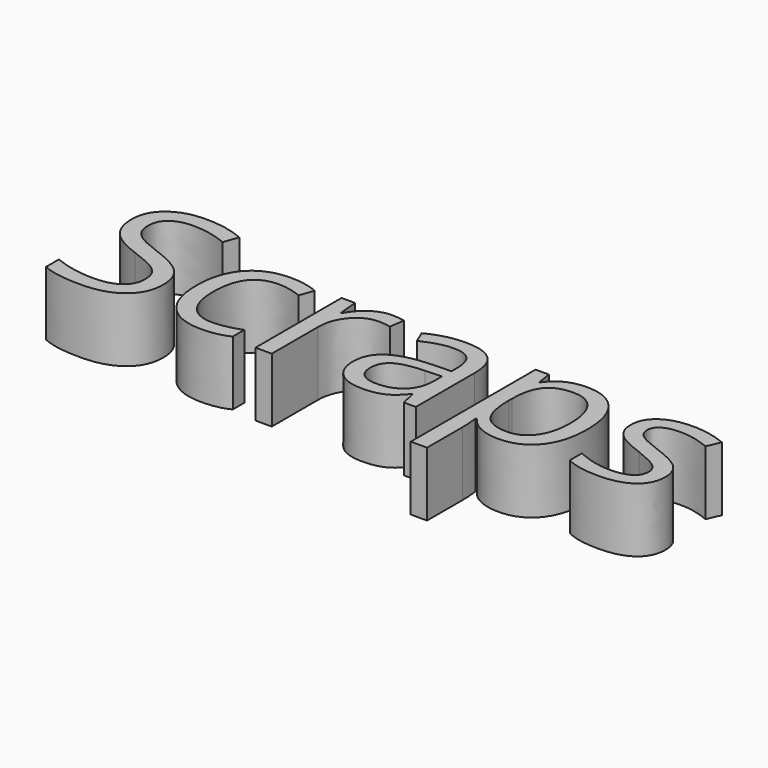
from build123d import *

# Parameters (mm, degrees)
F0_TEXT_SIZE = 17.2321063777
F1_DEPTH     = 5.5


# Not quite as in the source:
# - Text() gives the source's letters only with a copy of the font that has no kerning and outlines rounded to 1/6400 em; it was checked with that copy


with BuildPart() as f1:
    # F0 (on Top) → F1 (new body)
    with BuildSketch(Plane.XY):
        with Locations((-54.241374135, 26.8820896745)):
            Text('Scraps', F0_TEXT_SIZE, font='Open Sans', text_align=(TextAlign.LEFT, TextAlign.BOTTOM))
    extrude(amount=F1_DEPTH)


solid = f1.part
